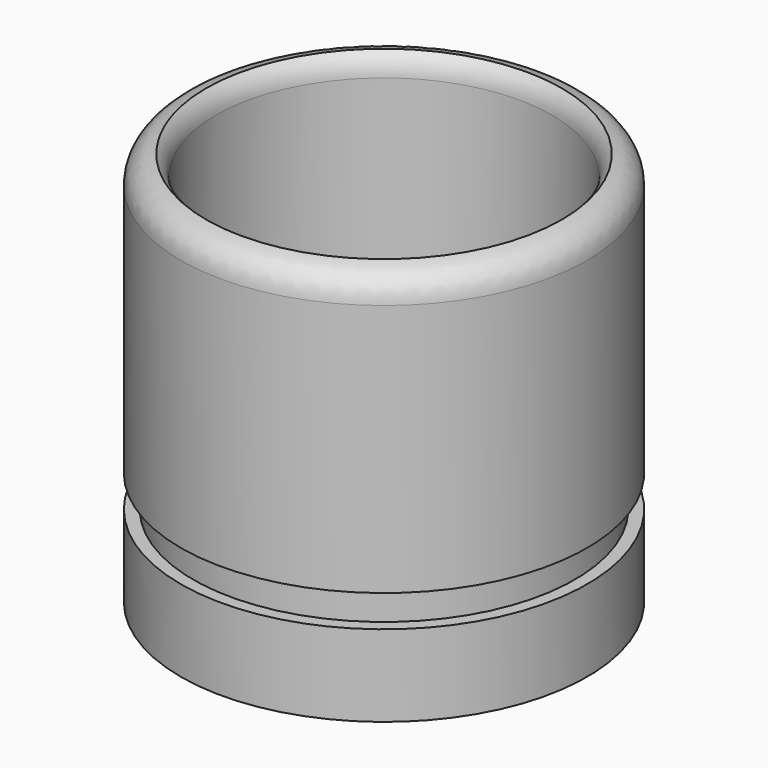
from build123d import *

# Parameters (mm, degrees)
F2_R = 5


# Not quite as in the source:
# - a fillet or chamfer that OpenCascade refuses, or shapes differently, is made with other operations: its cross-section is extruded or revolved along the edge and cut away or added


with BuildPart() as f1:
    # F0 (on Front) → F1 (revolve)
    with BuildSketch(Plane.XZ):
        Polygon((-30.2233248949, 37.0877869427), (-36.4803494329, 36.5061946213), (-36.4803494329, -13.4938053787), (-34.2613953475, -13.4938053787), (-34.2613953475, -19.2220297002), (-36.4803494329, -19.2220297002), (-36.4803494329, -33.86637941), (-19.9121574584, -33.86637941), (0, -33.86637941), (0, -26.3013252845), (-30.2233248949, -26.3013252845), align=None)
    revolve(axis=Axis((0, 0, -30.0838523473), (0, 0, 1)))

    # F2
    f2_edges = [f1.edges().sort_by_distance(p)[0] for p in [
        (36.480349, 0, 36.506195),
    ]]
    fillet(f2_edges, radius=F2_R)

    # F3: fillet of radius 5 on 2 edges, made by hand

    # F3_s1 → F3_t2 (revolve, cut)
    with BuildSketch(Plane.XZ):
        with BuildLine():
            ThreePointArc((-31.9428428579, 36.9282346211), (-30.6731716306, 35.2277917828), (-30.2229248949, 33.1539430061))
            Line((-30.2229248949, 33.1539430061), (-29.7228023494, 33.1539430061))
            ThreePointArc((-29.7228023494, 33.1539430061), (-29.7232023494, 35.1208649744), (-29.7232023494, 37.0877869427))
            Line((-29.7232023494, 37.0877869427), (-30.2696119123, 37.5857629186))
            ThreePointArc((-30.2696119123, 37.5857629186), (-31.1293581124, 37.5058492495), (-31.6147121087, 37.3056637826))
            Line((-31.6147121087, 37.3056637826), (-31.9428428579, 36.9282346211))
        make_face()
    revolve(axis=Axis((0, 0, 37.0877869427), (0, 0, 1)), mode=Mode.SUBTRACT)


solid = f1.part
